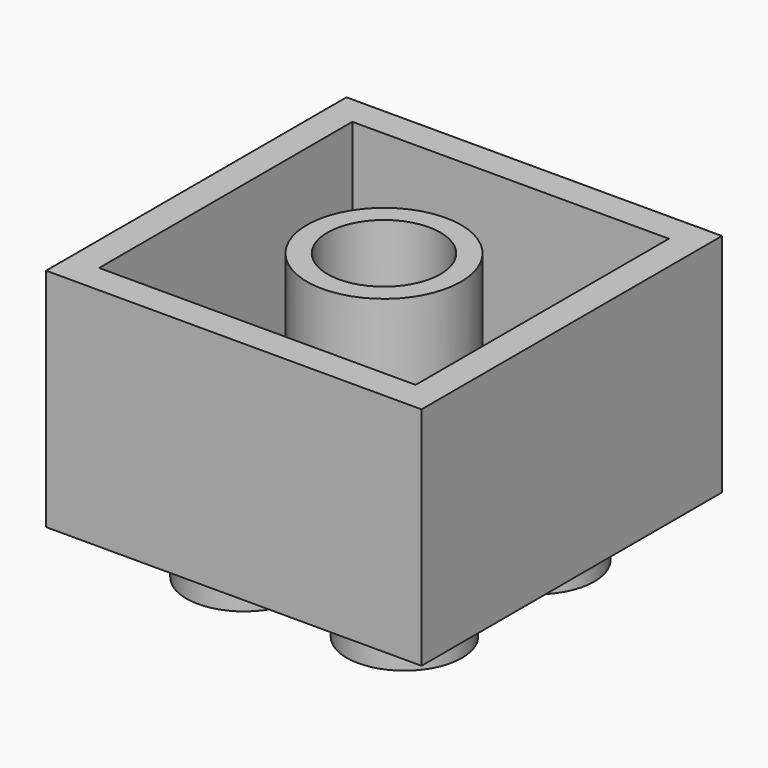
from build123d import *

# Parameters (mm, degrees)
F0_W     = 15.8
F0_H     = 15.8
F0_R     = 2.425
F1_DEPTH = 9.5
F2_DEPTH = 2.1
F3_W     = 13.32
F3_H     = 13.32
F3_R     = 3.24
F4_DEPTH = 8.76
F5_R     = 2.375
F6_DEPTH = 8.7


# Not quite as in the source:
# - a feature names something its author has since deleted; it is built from what else it names


with BuildPart() as f1:
    # F0 (on Top) → F1 (new body)
    with BuildSketch(Plane.XY):
        Rectangle(F0_W, F0_H)
        with Locations((-3.1053028645, -3.481)):
            Circle(F0_R, mode=Mode.SUBTRACT)
        with Locations((3.6446971353, -3.4810496163)):
            Circle(F0_R, mode=Mode.SUBTRACT)
        with Locations((-3.1053028647, 3.481)):
            Circle(F0_R, mode=Mode.SUBTRACT)
        with Locations((3.6446971353, 3.481)):
            Circle(F0_R, mode=Mode.SUBTRACT)
        with Locations((3.6446971353, -3.4810496163)):
            Circle(F0_R)
        with Locations((-3.1053028645, -3.481)):
            Circle(F0_R)
        with Locations((-3.1053028647, 3.481)):
            Circle(F0_R)
        with Locations((3.6446971353, 3.481)):
            Circle(F0_R)
    extrude(amount=F1_DEPTH)

    # F0 (on Top) → F2 (join)
    with BuildSketch(Plane.XY):
        with Locations((3.6446971353, 3.481)):
            Circle(F0_R)
        with Locations((-3.1053028647, 3.481)):
            Circle(F0_R)
        with Locations((-3.1053028645, -3.481)):
            Circle(F0_R)
        with Locations((3.6446971353, -3.4810496163)):
            Circle(F0_R)
    extrude(amount=-F2_DEPTH)

    # F3 (on face) → F4 (cut)
    with BuildSketch(Plane.XY.offset(9.5)):
        Rectangle(F3_W, F3_H)
        Circle(F3_R, mode=Mode.SUBTRACT)
    extrude(amount=-F4_DEPTH, mode=Mode.SUBTRACT)

    # F5 (on face) → F6 (cut)
    with BuildSketch(Plane.XY.offset(9.5)):
        Circle(F5_R)
    extrude(amount=-F6_DEPTH, mode=Mode.SUBTRACT)


solid = f1.part
